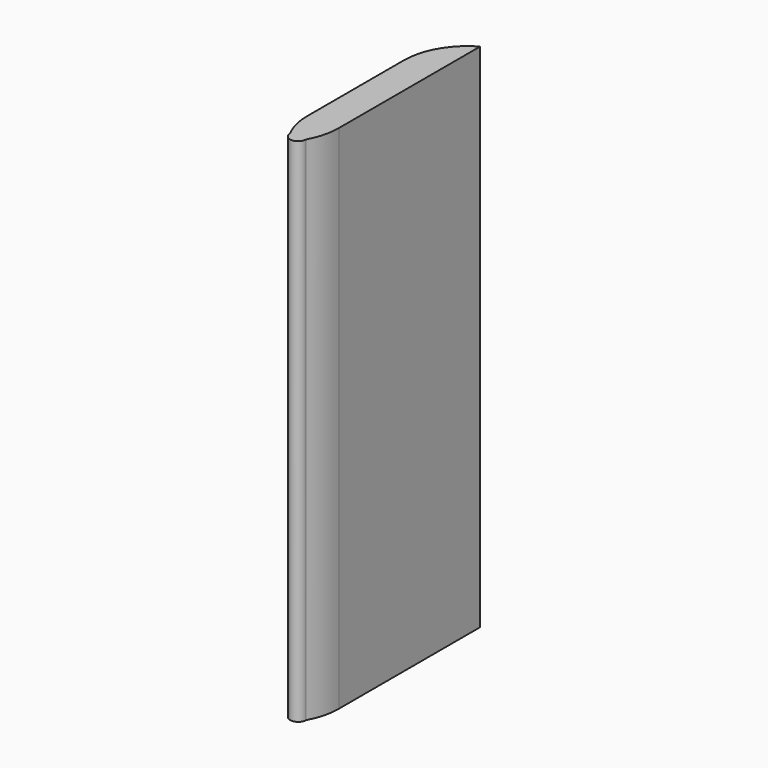
from build123d import *

# Parameters (mm, degrees)
F1_DEPTH    = 40.64
F2_T1_DEPTH = 62.6370452561
F3_T1_DEPTH = 52.9367221242


# Not quite as in the source:
# - a fillet or chamfer that OpenCascade refuses, or shapes differently, is made with other operations: its cross-section is extruded or revolved along the edge and cut away or added


with BuildPart() as f1:
    # F0 (on Top) → F1 (new body)
    with BuildSketch(Plane.XY):
        with BuildLine():
            Line((0.635, -8.255), (1.27, -8.255))
            Line((1.27, -8.255), (1.27, 8.255))
            Line((1.27, 8.255), (-1.27, 8.255))
            Line((-1.27, 8.255), (-1.27, -8.255))
            Line((-1.27, -8.255), (-0.635, -8.255))
            ThreePointArc((-0.635, -8.255), (0, -7.62), (0.635, -8.255))
        make_face()
        with BuildLine():
            ThreePointArc((-0.635, -8.255), (0, -8.89), (0.635, -8.255))
            Line((0.635, -8.255), (-0.635, -8.255))
        make_face()
        with BuildLine():
            Line((-0.635, -8.255), (0.635, -8.255))
            ThreePointArc((0.635, -8.255), (0, -7.62), (-0.635, -8.255))
        make_face()
    extrude(amount=F1_DEPTH)

    # F2: fillet of radius 5.08 on 1 edges, made by hand

    # F2_s2 → F2_t1 (cut)
    with BuildSketch(Plane.XY.offset(-10.9985226281)):
        with BuildLine():
            ThreePointArc((1.27, 8.255), (-0.5894090512, 6.3955909488), (-1.27, 3.8555909488))
            Line((-1.27, 3.8555909488), (-1.27, 8.255))
            Line((-1.27, 8.255), (1.27, 8.255))
        make_face()
    extrude(amount=F2_T1_DEPTH, mode=Mode.SUBTRACT)

    # F3: fillet of radius 5.08 on 2 edges, made by hand

    # F3_s2 → F3_t1 (cut)
    with BuildSketch(Plane.XY.offset(-6.1483610621)):
        with BuildLine():
            ThreePointArc((-0.635, -8.255), (-1.1086888497, -7.0656555752), (-1.27, -5.7956555752))
            Line((-1.27, -5.7956555752), (-1.27, -8.255))
            Line((-1.27, -8.255), (-0.635, -8.255))
        make_face()
        with BuildLine():
            ThreePointArc((0.635, -8.255), (1.1086888497, -7.0656555752), (1.27, -5.7956555752))
            Line((1.27, -5.7956555752), (1.27, -8.255))
            Line((1.27, -8.255), (0.635, -8.255))
        make_face()
    extrude(amount=F3_T1_DEPTH, mode=Mode.SUBTRACT)


solid = f1.part
